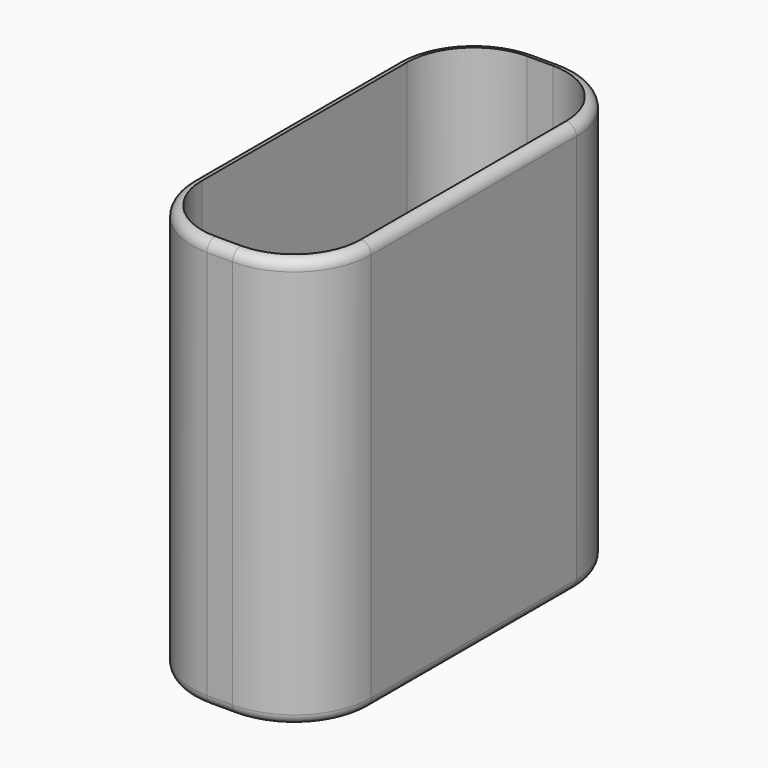
from build123d import *

# Parameters (mm, degrees)
F0_W     = 44.45
F0_H     = 101.6
F1_DEPTH = 101.6
F2_R     = 19.05
F3_T     = -2.54
F4_R     = 2.53999


# Not quite as in the source:
# - a fillet or chamfer is up to 0.001 mm smaller than in the source, because OpenCascade refuses the exact size


with BuildPart() as f1:
    # F0 (on Top) → F1 (new body)
    with BuildSketch(Plane.XY):
        Rectangle(F0_W, F0_H)
    extrude(amount=F1_DEPTH)

    # F2
    f2_edges = [f1.edges().sort_by_distance(p)[0] for p in [
        (-22.225, 50.8, 50.8),
        (-22.225, -50.8, 50.8),
        (22.225, -50.8, 50.8),
        (22.225, 50.8, 50.8),
    ]]
    fillet(f2_edges, radius=F2_R)

    # F3
    f3_openings = [f1.faces().sort_by_distance(p)[0] for p in [
        (0, 0, 101.6),
    ]]
    offset(amount=F3_T, openings=f3_openings)

    # F4 (radius 2.54 in the source; OpenCascade refuses exactly that, so slightly less here)
    f4_edges = [f1.edges().sort_by_distance(p)[0] for p in [
        (22.225, 0, 0),
        (22.225, -31.75, 50.8),
        (22.225, 31.75, 50.8),
        (22.225, 0, 101.6),
        (-22.225, 0, 0),
        (-22.225, 31.75, 50.8),
        (-22.225, -31.75, 50.8),
        (-22.225, 0, 101.6),
    ]]
    fillet(f4_edges, radius=F4_R)


solid = f1.part
